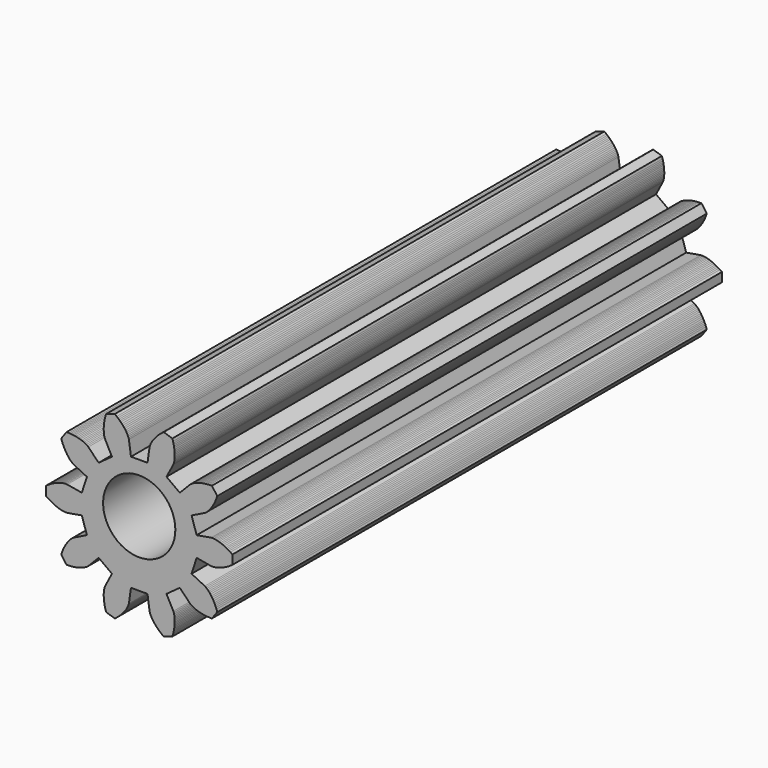
from build123d import *

# Parameters (mm, degrees)
F4_R     = 2.9504762809
F5_DEPTH = 250


# Not quite as in the source:
# - ends of sketch curves that miss each other by under 0.0002 mm in the source are joined


with BuildPart() as f3:
    # F0 (on Front) → F3 section 0
    with BuildSketch(Plane.XZ):
        with BuildLine():
            ThreePointArc((4.2753417889, -0.9237346066), (4.4837280553, -0.2822940953), (4.6921702972, 0.3591282284))
            Line((4.6921702972, 0.3591282284), (5.878934, 0.152889))
            Line((5.878934, 0.152889), (5.978914, 0.147897))
            Line((5.978914, 0.147897), (6.083031, 0.153397))
            Line((6.083031, 0.153397), (6.188792, 0.166293))
            Line((6.188792, 0.166293), (6.296123, 0.185564))
            Line((6.296123, 0.185564), (6.39688, 0.208667))
            Line((6.39688, 0.208667), (6.507485, 0.239158))
            Line((6.507485, 0.239158), (6.627466, 0.277934))
            Line((6.627466, 0.277934), (6.729844, 0.315505))
            Line((6.729844, 0.315505), (6.837582, 0.359366))
            Line((6.837582, 0.359366), (6.95036, 0.409935))
            Line((6.95036, 0.409935), (7.067828, 0.467611))
            Line((7.067828, 0.467611), (7.158791, 0.515766))
            Line((7.158791, 0.515766), (7.252025, 0.568292))
            Line((7.252025, 0.568292), (7.347362, 0.62534))
            Line((7.347362, 0.62534), (7.444626, 0.687056))
            Line((7.444626, 0.687056), (7.610854, 0.801339))
            Line((7.610854, 0.801339), (7.610854, 1.547781))
            Line((7.610854, 1.547781), (7.444624, 1.662064))
            Line((7.444624, 1.662064), (7.347361, 1.723779))
            Line((7.347361, 1.723779), (7.252025, 1.780827))
            Line((7.252025, 1.780827), (7.15879, 1.833354))
            Line((7.15879, 1.833354), (7.067828, 1.881508))
            Line((7.067828, 1.881508), (6.950358, 1.939185))
            Line((6.950358, 1.939185), (6.837582, 1.989753))
            Line((6.837582, 1.989753), (6.729843, 2.033614))
            Line((6.729843, 2.033614), (6.627464, 2.071186))
            Line((6.627464, 2.071186), (6.507485, 2.109962))
            Line((6.507485, 2.109962), (6.39688, 2.140452))
            Line((6.39688, 2.140452), (6.296123, 2.163555))
            Line((6.296123, 2.163555), (6.188792, 2.182826))
            Line((6.188792, 2.182826), (6.08303, 2.195722))
            Line((6.08303, 2.195722), (5.978914, 2.201222))
            Line((5.978914, 2.201222), (5.878933, 2.19623))
            Line((5.878933, 2.19623), (4.692172, 1.989989))
            ThreePointArc((4.692172, 1.989989), (4.4837309325, 2.6314120428), (4.2753451638, 3.2728530532))
            Line((4.2753451638, 3.2728530532), (5.35668, 3.80356))
            Line((5.35668, 3.80356), (5.4405, 3.858289))
            Line((5.4405, 3.858289), (5.5215, 3.923937))
            Line((5.5215, 3.923937), (5.599482, 3.996535))
            Line((5.599482, 3.996535), (5.674988, 4.075213))
            Line((5.674988, 4.075213), (5.742922, 4.153126))
            Line((5.742922, 4.153126), (5.814482, 4.242806))
            Line((5.814482, 4.242806), (5.888756, 4.344699))
            Line((5.888756, 4.344699), (5.949498, 4.435272))
            Line((5.949498, 4.435272), (6.010879, 4.534083))
            Line((6.010879, 4.534083), (6.072394, 4.641282))
            Line((6.072394, 4.641282), (6.133527, 4.75699))
            Line((6.133527, 4.75699), (6.178813, 4.849415))
            Line((6.178813, 4.849415), (6.223367, 4.946711))
            Line((6.223367, 4.946711), (6.266963, 5.048901))
            Line((6.266963, 5.048901), (6.309377, 5.156001))
            Line((6.309377, 5.156001), (6.376684, 5.346164))
            Line((6.376684, 5.346164), (5.937936, 5.950048))
            Line((5.937936, 5.950048), (5.73628, 5.944798))
            Line((5.73628, 5.944798), (5.621317, 5.937556))
            Line((5.621317, 5.937556), (5.510656, 5.927672))
            Line((5.510656, 5.927672), (5.404354, 5.915365))
            Line((5.404354, 5.915365), (5.302459, 5.900857))
            Line((5.302459, 5.900857), (5.173523, 5.878471))
            Line((5.173523, 5.878471), (5.052562, 5.853093))
            Line((5.052562, 5.853093), (4.939618, 5.825251))
            Line((4.939618, 5.825251), (4.834708, 5.79547))
            Line((4.834708, 5.79547), (4.714851, 5.756318))
            Line((4.714851, 5.756318), (4.607447, 5.715973))
            Line((4.607447, 5.715973), (4.512354, 5.67544))
            Line((4.512354, 5.67544), (4.414194, 5.627943))
            Line((4.414194, 5.627943), (4.321051, 5.576212))
            Line((4.321051, 5.576212), (4.233586, 5.519463))
            Line((4.233586, 5.519463), (4.155634, 5.456658))
            Line((4.155634, 5.456658), (3.31675, 4.592245))
            ThreePointArc((3.31675, 4.592245), (2.7710979645, 4.9886473644), (2.2254808469, 5.3850977893))
            Line((2.2254808469, 5.3850977893), (2.788358, 6.450042))
            Line((2.788358, 6.450042), (2.824001, 6.543587))
            Line((2.824001, 6.543587), (2.850944, 6.644307))
            Line((2.850944, 6.644307), (2.871361, 6.748877))
            Line((2.871361, 6.748877), (2.886201, 6.856911))
            Line((2.886201, 6.856911), (2.895364, 6.959874))
            Line((2.895364, 6.959874), (2.900545, 7.074489))
            Line((2.900545, 7.074489), (2.900742, 7.200579))
            Line((2.900742, 7.200579), (2.896647, 7.309556))
            Line((2.896647, 7.309556), (2.888225, 7.425575))
            Line((2.888225, 7.425575), (2.874982, 7.548459))
            Line((2.874982, 7.548459), (2.856428, 7.678002))
            Line((2.856428, 7.678002), (2.83874, 7.779394))
            Line((2.83874, 7.779394), (2.817595, 7.884296))
            Line((2.817595, 7.884296), (2.792799, 7.992596))
            Line((2.792799, 7.992596), (2.76416, 8.10417))
            Line((2.76416, 8.10417), (2.706839, 8.297578))
            Line((2.706839, 8.297578), (1.99693, 8.528241))
            Line((1.99693, 8.528241), (1.836873, 8.405463))
            Line((1.836873, 8.405463), (1.748122, 8.332031))
            Line((1.748122, 8.332031), (1.664405, 8.258989))
            Line((1.664405, 8.258989), (1.585639, 8.186549))
            Line((1.585639, 8.186549), (1.511732, 8.11492))
            Line((1.511732, 8.11492), (1.420578, 8.021022))
            Line((1.420578, 8.021022), (1.337635, 7.929392))
            Line((1.337635, 7.929392), (1.262627, 7.840481))
            Line((1.262627, 7.840481), (1.195258, 7.754723))
            Line((1.195258, 7.754723), (1.121305, 7.652599))
            Line((1.121305, 7.652599), (1.058128, 7.556829))
            Line((1.058128, 7.556829), (1.00502, 7.468143))
            Line((1.00502, 7.468143), (0.953525, 7.37202))
            Line((0.953525, 7.37202), (0.908577, 7.27542))
            Line((0.908577, 7.27542), (0.871173, 7.178099))
            Line((0.871173, 7.178099), (0.845025, 7.081469))
            Line((0.845025, 7.081469), (0.674443, 5.88906))
            ThreePointArc((0.674443, 5.88906), (1.5e-06, 5.8890320012), (-0.67444, 5.8890618078))
            Line((-0.67444, 5.8890618078), (-0.845022, 7.08147))
            Line((-0.845022, 7.08147), (-0.87117, 7.178099))
            Line((-0.87117, 7.178099), (-0.908574, 7.27542))
            Line((-0.908574, 7.27542), (-0.953521, 7.37202))
            Line((-0.953521, 7.37202), (-1.005016, 7.468143))
            Line((-1.005016, 7.468143), (-1.058124, 7.556829))
            Line((-1.058124, 7.556829), (-1.121301, 7.652598))
            Line((-1.121301, 7.652598), (-1.195255, 7.754725))
            Line((-1.195255, 7.754725), (-1.262624, 7.840481))
            Line((-1.262624, 7.840481), (-1.337632, 7.929392))
            Line((-1.337632, 7.929392), (-1.420575, 8.021024))
            Line((-1.420575, 8.021024), (-1.511728, 8.11492))
            Line((-1.511728, 8.11492), (-1.585636, 8.186551))
            Line((-1.585636, 8.186551), (-1.664402, 8.25899))
            Line((-1.664402, 8.25899), (-1.748119, 8.332032))
            Line((-1.748119, 8.332032), (-1.83687, 8.405464))
            Line((-1.83687, 8.405464), (-1.996926, 8.528241))
            Line((-1.996926, 8.528241), (-2.706835, 8.297578))
            Line((-2.706835, 8.297578), (-2.764157, 8.104169))
            Line((-2.764157, 8.104169), (-2.792795, 7.992595))
            Line((-2.792795, 7.992595), (-2.817591, 7.884296))
            Line((-2.817591, 7.884296), (-2.838736, 7.779392))
            Line((-2.838736, 7.779392), (-2.856425, 7.678002))
            Line((-2.856425, 7.678002), (-2.874978, 7.548459))
            Line((-2.874978, 7.548459), (-2.888221, 7.425576))
            Line((-2.888221, 7.425576), (-2.896643, 7.309556))
            Line((-2.896643, 7.309556), (-2.900739, 7.200578))
            Line((-2.900739, 7.200578), (-2.900542, 7.074489))
            Line((-2.900542, 7.074489), (-2.895361, 6.959875))
            Line((-2.895361, 6.959875), (-2.886197, 6.856911))
            Line((-2.886197, 6.856911), (-2.871358, 6.748877))
            Line((-2.871358, 6.748877), (-2.850941, 6.644307))
            Line((-2.850941, 6.644307), (-2.823998, 6.543587))
            Line((-2.823998, 6.543587), (-2.788355, 6.450042))
            Line((-2.788355, 6.450042), (-2.225478, 5.385097))
            ThreePointArc((-2.225478, 5.385097), (-2.771095971, 4.9886482498), (-3.3167477562, 4.592246041))
            Line((-3.3167477562, 4.592246041), (-4.155632, 5.456658))
            Line((-4.155632, 5.456658), (-4.233584, 5.519464))
            Line((-4.233584, 5.519464), (-4.321049, 5.576213))
            Line((-4.321049, 5.576213), (-4.414192, 5.627944))
            Line((-4.414192, 5.627944), (-4.512352, 5.675442))
            Line((-4.512352, 5.675442), (-4.607445, 5.715974))
            Line((-4.607445, 5.715974), (-4.714848, 5.756319))
            Line((-4.714848, 5.756319), (-4.834706, 5.795471))
            Line((-4.834706, 5.795471), (-4.939616, 5.825252))
            Line((-4.939616, 5.825252), (-5.052559, 5.853094))
            Line((-5.052559, 5.853094), (-5.173522, 5.878472))
            Line((-5.173522, 5.878472), (-5.302457, 5.900857))
            Line((-5.302457, 5.900857), (-5.404352, 5.915366))
            Line((-5.404352, 5.915366), (-5.510654, 5.927673))
            Line((-5.510654, 5.927673), (-5.621316, 5.937558))
            Line((-5.621316, 5.937558), (-5.736279, 5.944799))
            Line((-5.736279, 5.944799), (-5.937934, 5.950049))
            Line((-5.937934, 5.950049), (-6.376683, 5.346165))
            Line((-6.376683, 5.346165), (-6.309373, 5.156001))
            Line((-6.309373, 5.156001), (-6.266961, 5.048902))
            Line((-6.266961, 5.048902), (-6.223364, 4.946712))
            Line((-6.223364, 4.946712), (-6.17881, 4.849415))
            Line((-6.17881, 4.849415), (-6.133525, 4.756991))
            Line((-6.133525, 4.756991), (-6.072391, 4.641283))
            Line((-6.072391, 4.641283), (-6.010877, 4.534084))
            Line((-6.010877, 4.534084), (-5.949495, 4.435272))
            Line((-5.949495, 4.435272), (-5.888753, 4.344699))
            Line((-5.888753, 4.344699), (-5.81448, 4.242807))
            Line((-5.81448, 4.242807), (-5.74292, 4.153128))
            Line((-5.74292, 4.153128), (-5.674986, 4.075214))
            Line((-5.674986, 4.075214), (-5.59948, 3.996536))
            Line((-5.59948, 3.996536), (-5.521498, 3.923937))
            Line((-5.521498, 3.923937), (-5.440498, 3.85829))
            Line((-5.440498, 3.85829), (-5.356678, 3.803561))
            Line((-5.356678, 3.803561), (-4.275343, 3.272853))
            ThreePointArc((-4.275343, 3.272853), (-4.4837282639, 2.6314121631), (-4.6921703347, 1.9899897838))
            Line((-4.6921703347, 1.9899897838), (-5.878932, 2.196231))
            Line((-5.878932, 2.196231), (-5.978913, 2.201222))
            Line((-5.978913, 2.201222), (-6.08303, 2.195723))
            Line((-6.08303, 2.195723), (-6.188791, 2.182826))
            Line((-6.188791, 2.182826), (-6.296122, 2.163555))
            Line((-6.296122, 2.163555), (-6.396879, 2.140453))
            Line((-6.396879, 2.140453), (-6.507485, 2.109962))
            Line((-6.507485, 2.109962), (-6.627465, 2.071186))
            Line((-6.627465, 2.071186), (-6.729843, 2.033615))
            Line((-6.729843, 2.033615), (-6.837581, 1.989753))
            Line((-6.837581, 1.989753), (-6.950359, 1.939185))
            Line((-6.950359, 1.939185), (-7.067828, 1.881509))
            Line((-7.067828, 1.881509), (-7.158791, 1.833354))
            Line((-7.158791, 1.833354), (-7.252025, 1.780828))
            Line((-7.252025, 1.780828), (-7.347361, 1.723779))
            Line((-7.347361, 1.723779), (-7.444625, 1.662064))
            Line((-7.444625, 1.662064), (-7.610853, 1.547781))
            Line((-7.610853, 1.547781), (-7.610853, 0.801339))
            Line((-7.610853, 0.801339), (-7.444624, 0.687056))
            Line((-7.444624, 0.687056), (-7.34736, 0.625341))
            Line((-7.34736, 0.625341), (-7.252024, 0.568293))
            Line((-7.252024, 0.568293), (-7.158789, 0.515766))
            Line((-7.158789, 0.515766), (-7.067828, 0.467612))
            Line((-7.067828, 0.467612), (-6.950358, 0.409935))
            Line((-6.950358, 0.409935), (-6.837581, 0.359367))
            Line((-6.837581, 0.359367), (-6.729843, 0.315506))
            Line((-6.729843, 0.315506), (-6.627464, 0.277934))
            Line((-6.627464, 0.277934), (-6.507485, 0.239159))
            Line((-6.507485, 0.239159), (-6.396879, 0.208668))
            Line((-6.396879, 0.208668), (-6.296122, 0.185565))
            Line((-6.296122, 0.185565), (-6.18879, 0.166294))
            Line((-6.18879, 0.166294), (-6.083029, 0.153398))
            Line((-6.083029, 0.153398), (-5.978913, 0.147898))
            Line((-5.978913, 0.147898), (-5.878932, 0.15289))
            Line((-5.878932, 0.15289), (-4.692171, 0.359131))
            ThreePointArc((-4.692171, 0.359131), (-4.4837298858, -0.2822915276), (-4.2753442362, -0.9237320767))
            Line((-4.2753442362, -0.9237320767), (-5.356681, -1.45444))
            Line((-5.356681, -1.45444), (-5.440501, -1.509168))
            Line((-5.440501, -1.509168), (-5.5215, -1.574816))
            Line((-5.5215, -1.574816), (-5.599482, -1.647414))
            Line((-5.599482, -1.647414), (-5.674988, -1.726092))
            Line((-5.674988, -1.726092), (-5.742923, -1.804005))
            Line((-5.742923, -1.804005), (-5.814482, -1.893685))
            Line((-5.814482, -1.893685), (-5.888757, -1.995578))
            Line((-5.888757, -1.995578), (-5.949499, -2.08615))
            Line((-5.949499, -2.08615), (-6.010879, -2.184962))
            Line((-6.010879, -2.184962), (-6.072395, -2.292162))
            Line((-6.072395, -2.292162), (-6.133528, -2.407869))
            Line((-6.133528, -2.407869), (-6.178814, -2.500294))
            Line((-6.178814, -2.500294), (-6.223368, -2.59759))
            Line((-6.223368, -2.59759), (-6.266964, -2.69978))
            Line((-6.266964, -2.69978), (-6.309378, -2.80688))
            Line((-6.309378, -2.80688), (-6.376685, -2.997043))
            Line((-6.376685, -2.997043), (-5.937937, -3.600927))
            Line((-5.937937, -3.600927), (-5.736281, -3.595677))
            Line((-5.736281, -3.595677), (-5.621318, -3.588435))
            Line((-5.621318, -3.588435), (-5.510657, -3.578551))
            Line((-5.510657, -3.578551), (-5.404354, -3.566244))
            Line((-5.404354, -3.566244), (-5.30246, -3.551736))
            Line((-5.30246, -3.551736), (-5.173523, -3.52935))
            Line((-5.173523, -3.52935), (-5.052562, -3.503972))
            Line((-5.052562, -3.503972), (-4.939619, -3.47613))
            Line((-4.939619, -3.47613), (-4.834708, -3.446349))
            Line((-4.834708, -3.446349), (-4.714851, -3.407198))
            Line((-4.714851, -3.407198), (-4.607448, -3.366853))
            Line((-4.607448, -3.366853), (-4.512355, -3.32632))
            Line((-4.512355, -3.32632), (-4.414194, -3.278822))
            Line((-4.414194, -3.278822), (-4.321052, -3.227091))
            Line((-4.321052, -3.227091), (-4.233587, -3.170342))
            Line((-4.233587, -3.170342), (-4.155635, -3.107537))
            Line((-4.155635, -3.107537), (-3.31675, -2.243124))
            ThreePointArc((-3.31675, -2.243124), (-2.7710983472, -2.6395268912), (-2.2254812543, -3.0359773499))
            Line((-2.2254812543, -3.0359773499), (-2.788359, -4.100922))
            Line((-2.788359, -4.100922), (-2.824002, -4.194467))
            Line((-2.824002, -4.194467), (-2.850945, -4.295187))
            Line((-2.850945, -4.295187), (-2.871362, -4.399757))
            Line((-2.871362, -4.399757), (-2.886201, -4.50779))
            Line((-2.886201, -4.50779), (-2.895365, -4.610754))
            Line((-2.895365, -4.610754), (-2.900546, -4.725369))
            Line((-2.900546, -4.725369), (-2.900744, -4.851459))
            Line((-2.900744, -4.851459), (-2.896648, -4.960437))
            Line((-2.896648, -4.960437), (-2.888226, -5.076456))
            Line((-2.888226, -5.076456), (-2.874983, -5.19934))
            Line((-2.874983, -5.19934), (-2.856429, -5.328883))
            Line((-2.856429, -5.328883), (-2.838741, -5.430275))
            Line((-2.838741, -5.430275), (-2.817596, -5.535177))
            Line((-2.817596, -5.535177), (-2.7928, -5.643476))
            Line((-2.7928, -5.643476), (-2.764162, -5.75505))
            Line((-2.764162, -5.75505), (-2.70684, -5.948458))
            Line((-2.70684, -5.948458), (-1.996931, -6.179121))
            Line((-1.996931, -6.179121), (-1.836874, -6.056343))
            Line((-1.836874, -6.056343), (-1.748123, -5.982912))
            Line((-1.748123, -5.982912), (-1.664406, -5.90987))
            Line((-1.664406, -5.90987), (-1.585639, -5.83743))
            Line((-1.585639, -5.83743), (-1.511733, -5.765801))
            Line((-1.511733, -5.765801), (-1.420579, -5.671903))
            Line((-1.420579, -5.671903), (-1.337636, -5.580273))
            Line((-1.337636, -5.580273), (-1.262628, -5.491361))
            Line((-1.262628, -5.491361), (-1.195259, -5.405603))
            Line((-1.195259, -5.405603), (-1.121305, -5.303479))
            Line((-1.121305, -5.303479), (-1.058128, -5.207709))
            Line((-1.058128, -5.207709), (-1.00502, -5.119023))
            Line((-1.00502, -5.119023), (-0.953526, -5.0229))
            Line((-0.953526, -5.0229), (-0.908578, -4.9263))
            Line((-0.908578, -4.9263), (-0.871174, -4.828979))
            Line((-0.871174, -4.828979), (-0.845026, -4.73235))
            Line((-0.845026, -4.73235), (-0.674443, -3.539941))
            ThreePointArc((-0.674443, -3.539941), (-1.5e-06, -3.5399120003), (0.67444, -3.5399416176))
            Line((0.67444, -3.5399416176), (0.845021, -4.732351))
            Line((0.845021, -4.732351), (0.87117, -4.82898))
            Line((0.87117, -4.82898), (0.908574, -4.926302))
            Line((0.908574, -4.926302), (0.953521, -5.022901))
            Line((0.953521, -5.022901), (1.005016, -5.119024))
            Line((1.005016, -5.119024), (1.058123, -5.20771))
            Line((1.058123, -5.20771), (1.1213, -5.30348))
            Line((1.1213, -5.30348), (1.195254, -5.405606))
            Line((1.195254, -5.405606), (1.262623, -5.491364))
            Line((1.262623, -5.491364), (1.337631, -5.580275))
            Line((1.337631, -5.580275), (1.420574, -5.671906))
            Line((1.420574, -5.671906), (1.511728, -5.765803))
            Line((1.511728, -5.765803), (1.585635, -5.837433))
            Line((1.585635, -5.837433), (1.664401, -5.909872))
            Line((1.664401, -5.909872), (1.748118, -5.982913))
            Line((1.748118, -5.982913), (1.836869, -6.056346))
            Line((1.836869, -6.056346), (1.996925, -6.179123))
            Line((1.996925, -6.179123), (2.706834, -5.94846))
            Line((2.706834, -5.94846), (2.764156, -5.755051))
            Line((2.764156, -5.755051), (2.792795, -5.643476))
            Line((2.792795, -5.643476), (2.817591, -5.535178))
            Line((2.817591, -5.535178), (2.838735, -5.430275))
            Line((2.838735, -5.430275), (2.856424, -5.328885))
            Line((2.856424, -5.328885), (2.874977, -5.199341))
            Line((2.874977, -5.199341), (2.888221, -5.076458))
            Line((2.888221, -5.076458), (2.896643, -4.960438))
            Line((2.896643, -4.960438), (2.900738, -4.851459))
            Line((2.900738, -4.851459), (2.900541, -4.725371))
            Line((2.900541, -4.725371), (2.89536, -4.610756))
            Line((2.89536, -4.610756), (2.886197, -4.507792))
            Line((2.886197, -4.507792), (2.871357, -4.399759))
            Line((2.871357, -4.399759), (2.850941, -4.295188))
            Line((2.850941, -4.295188), (2.823998, -4.194468))
            Line((2.823998, -4.194468), (2.788354, -4.100924))
            Line((2.788354, -4.100924), (2.225479, -3.035979))
            ThreePointArc((2.225479, -3.035979), (2.7710963565, -2.6395289039), (3.3167481995, -2.2431262746))
            Line((3.3167481995, -2.2431262746), (4.155631, -3.10754))
            Line((4.155631, -3.10754), (4.233583, -3.170346))
            Line((4.233583, -3.170346), (4.321048, -3.227095))
            Line((4.321048, -3.227095), (4.41419, -3.278826))
            Line((4.41419, -3.278826), (4.51235, -3.326324))
            Line((4.51235, -3.326324), (4.607444, -3.366856))
            Line((4.607444, -3.366856), (4.714847, -3.407201))
            Line((4.714847, -3.407201), (4.834705, -3.446354))
            Line((4.834705, -3.446354), (4.939615, -3.476134))
            Line((4.939615, -3.476134), (5.052558, -3.503976))
            Line((5.052558, -3.503976), (5.17352, -3.529355))
            Line((5.17352, -3.529355), (5.302456, -3.55174))
            Line((5.302456, -3.55174), (5.404351, -3.566249))
            Line((5.404351, -3.566249), (5.510653, -3.578556))
            Line((5.510653, -3.578556), (5.621314, -3.58844))
            Line((5.621314, -3.58844), (5.736278, -3.595682))
            Line((5.736278, -3.595682), (5.937933, -3.600932))
            Line((5.937933, -3.600932), (6.376681, -2.997048))
            Line((6.376681, -2.997048), (6.309372, -2.806883))
            Line((6.309372, -2.806883), (6.26696, -2.699785))
            Line((6.26696, -2.699785), (6.223363, -2.597595))
            Line((6.223363, -2.597595), (6.178809, -2.500297))
            Line((6.178809, -2.500297), (6.133524, -2.407874))
            Line((6.133524, -2.407874), (6.07239, -2.292165))
            Line((6.07239, -2.292165), (6.010875, -2.184966))
            Line((6.010875, -2.184966), (5.949495, -2.086155))
            Line((5.949495, -2.086155), (5.888752, -1.995582))
            Line((5.888752, -1.995582), (5.814479, -1.89369))
            Line((5.814479, -1.89369), (5.742919, -1.80401))
            Line((5.742919, -1.80401), (5.674985, -1.726096))
            Line((5.674985, -1.726096), (5.599479, -1.647418))
            Line((5.599479, -1.647418), (5.521497, -1.574819))
            Line((5.521497, -1.574819), (5.440498, -1.509172))
            Line((5.440498, -1.509172), (5.356677, -1.454443))
            Line((5.356677, -1.454443), (4.2753417889, -0.9237346066))
        make_face()
    # F2 (on offset) → F3 section 1
    with BuildSketch(Plane.XZ.offset(50)):
        with BuildLine():
            ThreePointArc((4.2753417889, -0.9237346066), (4.4837280553, -0.2822940953), (4.6921702972, 0.3591282284))
            Line((4.6921702972, 0.3591282284), (5.878934, 0.152889))
            Line((5.878934, 0.152889), (5.978914, 0.147897))
            Line((5.978914, 0.147897), (6.083031, 0.153397))
            Line((6.083031, 0.153397), (6.188792, 0.166293))
            Line((6.188792, 0.166293), (6.296123, 0.185564))
            Line((6.296123, 0.185564), (6.39688, 0.208667))
            Line((6.39688, 0.208667), (6.507485, 0.239158))
            Line((6.507485, 0.239158), (6.627466, 0.277934))
            Line((6.627466, 0.277934), (6.729844, 0.315505))
            Line((6.729844, 0.315505), (6.837582, 0.359366))
            Line((6.837582, 0.359366), (6.95036, 0.409935))
            Line((6.95036, 0.409935), (7.067828, 0.467611))
            Line((7.067828, 0.467611), (7.158791, 0.515766))
            Line((7.158791, 0.515766), (7.252025, 0.568292))
            Line((7.252025, 0.568292), (7.347362, 0.62534))
            Line((7.347362, 0.62534), (7.444626, 0.687056))
            Line((7.444626, 0.687056), (7.610854, 0.801339))
            Line((7.610854, 0.801339), (7.610854, 1.547781))
            Line((7.610854, 1.547781), (7.444624, 1.662064))
            Line((7.444624, 1.662064), (7.347361, 1.723779))
            Line((7.347361, 1.723779), (7.252025, 1.780827))
            Line((7.252025, 1.780827), (7.15879, 1.833354))
            Line((7.15879, 1.833354), (7.067828, 1.881508))
            Line((7.067828, 1.881508), (6.950358, 1.939185))
            Line((6.950358, 1.939185), (6.837582, 1.989753))
            Line((6.837582, 1.989753), (6.729843, 2.033614))
            Line((6.729843, 2.033614), (6.627464, 2.071186))
            Line((6.627464, 2.071186), (6.507485, 2.109962))
            Line((6.507485, 2.109962), (6.39688, 2.140452))
            Line((6.39688, 2.140452), (6.296123, 2.163555))
            Line((6.296123, 2.163555), (6.188792, 2.182826))
            Line((6.188792, 2.182826), (6.08303, 2.195722))
            Line((6.08303, 2.195722), (5.978914, 2.201222))
            Line((5.978914, 2.201222), (5.878933, 2.19623))
            Line((5.878933, 2.19623), (4.692172, 1.989989))
            ThreePointArc((4.692172, 1.989989), (4.4837309325, 2.6314120428), (4.2753451638, 3.2728530532))
            Line((4.2753451638, 3.2728530532), (5.35668, 3.80356))
            Line((5.35668, 3.80356), (5.4405, 3.858289))
            Line((5.4405, 3.858289), (5.5215, 3.923937))
            Line((5.5215, 3.923937), (5.599482, 3.996535))
            Line((5.599482, 3.996535), (5.674988, 4.075213))
            Line((5.674988, 4.075213), (5.742922, 4.153126))
            Line((5.742922, 4.153126), (5.814482, 4.242806))
            Line((5.814482, 4.242806), (5.888756, 4.344699))
            Line((5.888756, 4.344699), (5.949498, 4.435272))
            Line((5.949498, 4.435272), (6.010879, 4.534083))
            Line((6.010879, 4.534083), (6.072394, 4.641282))
            Line((6.072394, 4.641282), (6.133527, 4.75699))
            Line((6.133527, 4.75699), (6.178813, 4.849415))
            Line((6.178813, 4.849415), (6.223367, 4.946711))
            Line((6.223367, 4.946711), (6.266963, 5.048901))
            Line((6.266963, 5.048901), (6.309377, 5.156001))
            Line((6.309377, 5.156001), (6.376684, 5.346164))
            Line((6.376684, 5.346164), (5.937936, 5.950048))
            Line((5.937936, 5.950048), (5.73628, 5.944798))
            Line((5.73628, 5.944798), (5.621317, 5.937556))
            Line((5.621317, 5.937556), (5.510656, 5.927672))
            Line((5.510656, 5.927672), (5.404354, 5.915365))
            Line((5.404354, 5.915365), (5.302459, 5.900857))
            Line((5.302459, 5.900857), (5.173523, 5.878471))
            Line((5.173523, 5.878471), (5.052562, 5.853093))
            Line((5.052562, 5.853093), (4.939618, 5.825251))
            Line((4.939618, 5.825251), (4.834708, 5.79547))
            Line((4.834708, 5.79547), (4.714851, 5.756318))
            Line((4.714851, 5.756318), (4.607447, 5.715973))
            Line((4.607447, 5.715973), (4.512354, 5.67544))
            Line((4.512354, 5.67544), (4.414194, 5.627943))
            Line((4.414194, 5.627943), (4.321051, 5.576212))
            Line((4.321051, 5.576212), (4.233586, 5.519463))
            Line((4.233586, 5.519463), (4.155634, 5.456658))
            Line((4.155634, 5.456658), (3.31675, 4.592245))
            ThreePointArc((3.31675, 4.592245), (2.7710979645, 4.9886473644), (2.2254808469, 5.3850977893))
            Line((2.2254808469, 5.3850977893), (2.788358, 6.450042))
            Line((2.788358, 6.450042), (2.824001, 6.543587))
            Line((2.824001, 6.543587), (2.850944, 6.644307))
            Line((2.850944, 6.644307), (2.871361, 6.748877))
            Line((2.871361, 6.748877), (2.886201, 6.856911))
            Line((2.886201, 6.856911), (2.895364, 6.959874))
            Line((2.895364, 6.959874), (2.900545, 7.074489))
            Line((2.900545, 7.074489), (2.900742, 7.200579))
            Line((2.900742, 7.200579), (2.896647, 7.309556))
            Line((2.896647, 7.309556), (2.888225, 7.425575))
            Line((2.888225, 7.425575), (2.874982, 7.548459))
            Line((2.874982, 7.548459), (2.856428, 7.678002))
            Line((2.856428, 7.678002), (2.83874, 7.779394))
            Line((2.83874, 7.779394), (2.817595, 7.884296))
            Line((2.817595, 7.884296), (2.792799, 7.992596))
            Line((2.792799, 7.992596), (2.76416, 8.10417))
            Line((2.76416, 8.10417), (2.706839, 8.297578))
            Line((2.706839, 8.297578), (1.99693, 8.528241))
            Line((1.99693, 8.528241), (1.836873, 8.405463))
            Line((1.836873, 8.405463), (1.748122, 8.332031))
            Line((1.748122, 8.332031), (1.664405, 8.258989))
            Line((1.664405, 8.258989), (1.585639, 8.186549))
            Line((1.585639, 8.186549), (1.511732, 8.11492))
            Line((1.511732, 8.11492), (1.420578, 8.021022))
            Line((1.420578, 8.021022), (1.337635, 7.929392))
            Line((1.337635, 7.929392), (1.262627, 7.840481))
            Line((1.262627, 7.840481), (1.195258, 7.754723))
            Line((1.195258, 7.754723), (1.121305, 7.652599))
            Line((1.121305, 7.652599), (1.058128, 7.556829))
            Line((1.058128, 7.556829), (1.00502, 7.468143))
            Line((1.00502, 7.468143), (0.953525, 7.37202))
            Line((0.953525, 7.37202), (0.908577, 7.27542))
            Line((0.908577, 7.27542), (0.871173, 7.178099))
            Line((0.871173, 7.178099), (0.845025, 7.081469))
            Line((0.845025, 7.081469), (0.674443, 5.88906))
            ThreePointArc((0.674443, 5.88906), (1.5e-06, 5.8890320012), (-0.67444, 5.8890618078))
            Line((-0.67444, 5.8890618078), (-0.845022, 7.08147))
            Line((-0.845022, 7.08147), (-0.87117, 7.178099))
            Line((-0.87117, 7.178099), (-0.908574, 7.27542))
            Line((-0.908574, 7.27542), (-0.953521, 7.37202))
            Line((-0.953521, 7.37202), (-1.005016, 7.468143))
            Line((-1.005016, 7.468143), (-1.058124, 7.556829))
            Line((-1.058124, 7.556829), (-1.121301, 7.652598))
            Line((-1.121301, 7.652598), (-1.195255, 7.754725))
            Line((-1.195255, 7.754725), (-1.262624, 7.840481))
            Line((-1.262624, 7.840481), (-1.337632, 7.929392))
            Line((-1.337632, 7.929392), (-1.420575, 8.021024))
            Line((-1.420575, 8.021024), (-1.511728, 8.11492))
            Line((-1.511728, 8.11492), (-1.585636, 8.186551))
            Line((-1.585636, 8.186551), (-1.664402, 8.25899))
            Line((-1.664402, 8.25899), (-1.748119, 8.332032))
            Line((-1.748119, 8.332032), (-1.83687, 8.405464))
            Line((-1.83687, 8.405464), (-1.996926, 8.528241))
            Line((-1.996926, 8.528241), (-2.706835, 8.297578))
            Line((-2.706835, 8.297578), (-2.764157, 8.104169))
            Line((-2.764157, 8.104169), (-2.792795, 7.992595))
            Line((-2.792795, 7.992595), (-2.817591, 7.884296))
            Line((-2.817591, 7.884296), (-2.838736, 7.779392))
            Line((-2.838736, 7.779392), (-2.856425, 7.678002))
            Line((-2.856425, 7.678002), (-2.874978, 7.548459))
            Line((-2.874978, 7.548459), (-2.888221, 7.425576))
            Line((-2.888221, 7.425576), (-2.896643, 7.309556))
            Line((-2.896643, 7.309556), (-2.900739, 7.200578))
            Line((-2.900739, 7.200578), (-2.900542, 7.074489))
            Line((-2.900542, 7.074489), (-2.895361, 6.959875))
            Line((-2.895361, 6.959875), (-2.886197, 6.856911))
            Line((-2.886197, 6.856911), (-2.871358, 6.748877))
            Line((-2.871358, 6.748877), (-2.850941, 6.644307))
            Line((-2.850941, 6.644307), (-2.823998, 6.543587))
            Line((-2.823998, 6.543587), (-2.788355, 6.450042))
            Line((-2.788355, 6.450042), (-2.225478, 5.385097))
            ThreePointArc((-2.225478, 5.385097), (-2.771095971, 4.9886482498), (-3.3167477562, 4.592246041))
            Line((-3.3167477562, 4.592246041), (-4.155632, 5.456658))
            Line((-4.155632, 5.456658), (-4.233584, 5.519464))
            Line((-4.233584, 5.519464), (-4.321049, 5.576213))
            Line((-4.321049, 5.576213), (-4.414192, 5.627944))
            Line((-4.414192, 5.627944), (-4.512352, 5.675442))
            Line((-4.512352, 5.675442), (-4.607445, 5.715974))
            Line((-4.607445, 5.715974), (-4.714848, 5.756319))
            Line((-4.714848, 5.756319), (-4.834706, 5.795471))
            Line((-4.834706, 5.795471), (-4.939616, 5.825252))
            Line((-4.939616, 5.825252), (-5.052559, 5.853094))
            Line((-5.052559, 5.853094), (-5.173522, 5.878472))
            Line((-5.173522, 5.878472), (-5.302457, 5.900857))
            Line((-5.302457, 5.900857), (-5.404352, 5.915366))
            Line((-5.404352, 5.915366), (-5.510654, 5.927673))
            Line((-5.510654, 5.927673), (-5.621316, 5.937558))
            Line((-5.621316, 5.937558), (-5.736279, 5.944799))
            Line((-5.736279, 5.944799), (-5.937934, 5.950049))
            Line((-5.937934, 5.950049), (-6.376683, 5.346165))
            Line((-6.376683, 5.346165), (-6.309373, 5.156001))
            Line((-6.309373, 5.156001), (-6.266961, 5.048902))
            Line((-6.266961, 5.048902), (-6.223364, 4.946712))
            Line((-6.223364, 4.946712), (-6.17881, 4.849415))
            Line((-6.17881, 4.849415), (-6.133525, 4.756991))
            Line((-6.133525, 4.756991), (-6.072391, 4.641283))
            Line((-6.072391, 4.641283), (-6.010877, 4.534084))
            Line((-6.010877, 4.534084), (-5.949495, 4.435272))
            Line((-5.949495, 4.435272), (-5.888753, 4.344699))
            Line((-5.888753, 4.344699), (-5.81448, 4.242807))
            Line((-5.81448, 4.242807), (-5.74292, 4.153128))
            Line((-5.74292, 4.153128), (-5.674986, 4.075214))
            Line((-5.674986, 4.075214), (-5.59948, 3.996536))
            Line((-5.59948, 3.996536), (-5.521498, 3.923937))
            Line((-5.521498, 3.923937), (-5.440498, 3.85829))
            Line((-5.440498, 3.85829), (-5.356678, 3.803561))
            Line((-5.356678, 3.803561), (-4.275343, 3.272853))
            ThreePointArc((-4.275343, 3.272853), (-4.4837282639, 2.6314121631), (-4.6921703347, 1.9899897838))
            Line((-4.6921703347, 1.9899897838), (-5.878932, 2.196231))
            Line((-5.878932, 2.196231), (-5.978913, 2.201222))
            Line((-5.978913, 2.201222), (-6.08303, 2.195723))
            Line((-6.08303, 2.195723), (-6.188791, 2.182826))
            Line((-6.188791, 2.182826), (-6.296122, 2.163555))
            Line((-6.296122, 2.163555), (-6.396879, 2.140453))
            Line((-6.396879, 2.140453), (-6.507485, 2.109962))
            Line((-6.507485, 2.109962), (-6.627465, 2.071186))
            Line((-6.627465, 2.071186), (-6.729843, 2.033615))
            Line((-6.729843, 2.033615), (-6.837581, 1.989753))
            Line((-6.837581, 1.989753), (-6.950359, 1.939185))
            Line((-6.950359, 1.939185), (-7.067828, 1.881509))
            Line((-7.067828, 1.881509), (-7.158791, 1.833354))
            Line((-7.158791, 1.833354), (-7.252025, 1.780828))
            Line((-7.252025, 1.780828), (-7.347361, 1.723779))
            Line((-7.347361, 1.723779), (-7.444625, 1.662064))
            Line((-7.444625, 1.662064), (-7.610853, 1.547781))
            Line((-7.610853, 1.547781), (-7.610853, 0.801339))
            Line((-7.610853, 0.801339), (-7.444624, 0.687056))
            Line((-7.444624, 0.687056), (-7.34736, 0.625341))
            Line((-7.34736, 0.625341), (-7.252024, 0.568293))
            Line((-7.252024, 0.568293), (-7.158789, 0.515766))
            Line((-7.158789, 0.515766), (-7.067828, 0.467612))
            Line((-7.067828, 0.467612), (-6.950358, 0.409935))
            Line((-6.950358, 0.409935), (-6.837581, 0.359367))
            Line((-6.837581, 0.359367), (-6.729843, 0.315506))
            Line((-6.729843, 0.315506), (-6.627464, 0.277934))
            Line((-6.627464, 0.277934), (-6.507485, 0.239159))
            Line((-6.507485, 0.239159), (-6.396879, 0.208668))
            Line((-6.396879, 0.208668), (-6.296122, 0.185565))
            Line((-6.296122, 0.185565), (-6.18879, 0.166294))
            Line((-6.18879, 0.166294), (-6.083029, 0.153398))
            Line((-6.083029, 0.153398), (-5.978913, 0.147898))
            Line((-5.978913, 0.147898), (-5.878932, 0.15289))
            Line((-5.878932, 0.15289), (-4.692171, 0.359131))
            ThreePointArc((-4.692171, 0.359131), (-4.4837298858, -0.2822915276), (-4.2753442362, -0.9237320767))
            Line((-4.2753442362, -0.9237320767), (-5.356681, -1.45444))
            Line((-5.356681, -1.45444), (-5.440501, -1.509168))
            Line((-5.440501, -1.509168), (-5.5215, -1.574816))
            Line((-5.5215, -1.574816), (-5.599482, -1.647414))
            Line((-5.599482, -1.647414), (-5.674988, -1.726092))
            Line((-5.674988, -1.726092), (-5.742923, -1.804005))
            Line((-5.742923, -1.804005), (-5.814482, -1.893685))
            Line((-5.814482, -1.893685), (-5.888757, -1.995578))
            Line((-5.888757, -1.995578), (-5.949499, -2.08615))
            Line((-5.949499, -2.08615), (-6.010879, -2.184962))
            Line((-6.010879, -2.184962), (-6.072395, -2.292162))
            Line((-6.072395, -2.292162), (-6.133528, -2.407869))
            Line((-6.133528, -2.407869), (-6.178814, -2.500294))
            Line((-6.178814, -2.500294), (-6.223368, -2.59759))
            Line((-6.223368, -2.59759), (-6.266964, -2.69978))
            Line((-6.266964, -2.69978), (-6.309378, -2.80688))
            Line((-6.309378, -2.80688), (-6.376685, -2.997043))
            Line((-6.376685, -2.997043), (-5.937937, -3.600927))
            Line((-5.937937, -3.600927), (-5.736281, -3.595677))
            Line((-5.736281, -3.595677), (-5.621318, -3.588435))
            Line((-5.621318, -3.588435), (-5.510657, -3.578551))
            Line((-5.510657, -3.578551), (-5.404354, -3.566244))
            Line((-5.404354, -3.566244), (-5.30246, -3.551736))
            Line((-5.30246, -3.551736), (-5.173523, -3.52935))
            Line((-5.173523, -3.52935), (-5.052562, -3.503972))
            Line((-5.052562, -3.503972), (-4.939619, -3.47613))
            Line((-4.939619, -3.47613), (-4.834708, -3.446349))
            Line((-4.834708, -3.446349), (-4.714851, -3.407198))
            Line((-4.714851, -3.407198), (-4.607448, -3.366853))
            Line((-4.607448, -3.366853), (-4.512355, -3.32632))
            Line((-4.512355, -3.32632), (-4.414194, -3.278822))
            Line((-4.414194, -3.278822), (-4.321052, -3.227091))
            Line((-4.321052, -3.227091), (-4.233587, -3.170342))
            Line((-4.233587, -3.170342), (-4.155635, -3.107537))
            Line((-4.155635, -3.107537), (-3.31675, -2.243124))
            ThreePointArc((-3.31675, -2.243124), (-2.7710983472, -2.6395268912), (-2.2254812543, -3.0359773499))
            Line((-2.2254812543, -3.0359773499), (-2.788359, -4.100922))
            Line((-2.788359, -4.100922), (-2.824002, -4.194467))
            Line((-2.824002, -4.194467), (-2.850945, -4.295187))
            Line((-2.850945, -4.295187), (-2.871362, -4.399757))
            Line((-2.871362, -4.399757), (-2.886201, -4.50779))
            Line((-2.886201, -4.50779), (-2.895365, -4.610754))
            Line((-2.895365, -4.610754), (-2.900546, -4.725369))
            Line((-2.900546, -4.725369), (-2.900744, -4.851459))
            Line((-2.900744, -4.851459), (-2.896648, -4.960437))
            Line((-2.896648, -4.960437), (-2.888226, -5.076456))
            Line((-2.888226, -5.076456), (-2.874983, -5.19934))
            Line((-2.874983, -5.19934), (-2.856429, -5.328883))
            Line((-2.856429, -5.328883), (-2.838741, -5.430275))
            Line((-2.838741, -5.430275), (-2.817596, -5.535177))
            Line((-2.817596, -5.535177), (-2.7928, -5.643476))
            Line((-2.7928, -5.643476), (-2.764162, -5.75505))
            Line((-2.764162, -5.75505), (-2.70684, -5.948458))
            Line((-2.70684, -5.948458), (-1.996931, -6.179121))
            Line((-1.996931, -6.179121), (-1.836874, -6.056343))
            Line((-1.836874, -6.056343), (-1.748123, -5.982912))
            Line((-1.748123, -5.982912), (-1.664406, -5.90987))
            Line((-1.664406, -5.90987), (-1.585639, -5.83743))
            Line((-1.585639, -5.83743), (-1.511733, -5.765801))
            Line((-1.511733, -5.765801), (-1.420579, -5.671903))
            Line((-1.420579, -5.671903), (-1.337636, -5.580273))
            Line((-1.337636, -5.580273), (-1.262628, -5.491361))
            Line((-1.262628, -5.491361), (-1.195259, -5.405603))
            Line((-1.195259, -5.405603), (-1.121305, -5.303479))
            Line((-1.121305, -5.303479), (-1.058128, -5.207709))
            Line((-1.058128, -5.207709), (-1.00502, -5.119023))
            Line((-1.00502, -5.119023), (-0.953526, -5.0229))
            Line((-0.953526, -5.0229), (-0.908578, -4.9263))
            Line((-0.908578, -4.9263), (-0.871174, -4.828979))
            Line((-0.871174, -4.828979), (-0.845026, -4.73235))
            Line((-0.845026, -4.73235), (-0.674443, -3.539941))
            ThreePointArc((-0.674443, -3.539941), (-1.5e-06, -3.5399120003), (0.67444, -3.5399416176))
            Line((0.67444, -3.5399416176), (0.845021, -4.732351))
            Line((0.845021, -4.732351), (0.87117, -4.82898))
            Line((0.87117, -4.82898), (0.908574, -4.926302))
            Line((0.908574, -4.926302), (0.953521, -5.022901))
            Line((0.953521, -5.022901), (1.005016, -5.119024))
            Line((1.005016, -5.119024), (1.058123, -5.20771))
            Line((1.058123, -5.20771), (1.1213, -5.30348))
            Line((1.1213, -5.30348), (1.195254, -5.405606))
            Line((1.195254, -5.405606), (1.262623, -5.491364))
            Line((1.262623, -5.491364), (1.337631, -5.580275))
            Line((1.337631, -5.580275), (1.420574, -5.671906))
            Line((1.420574, -5.671906), (1.511728, -5.765803))
            Line((1.511728, -5.765803), (1.585635, -5.837433))
            Line((1.585635, -5.837433), (1.664401, -5.909872))
            Line((1.664401, -5.909872), (1.748118, -5.982913))
            Line((1.748118, -5.982913), (1.836869, -6.056346))
            Line((1.836869, -6.056346), (1.996925, -6.179123))
            Line((1.996925, -6.179123), (2.706834, -5.94846))
            Line((2.706834, -5.94846), (2.764156, -5.755051))
            Line((2.764156, -5.755051), (2.792795, -5.643476))
            Line((2.792795, -5.643476), (2.817591, -5.535178))
            Line((2.817591, -5.535178), (2.838735, -5.430275))
            Line((2.838735, -5.430275), (2.856424, -5.328885))
            Line((2.856424, -5.328885), (2.874977, -5.199341))
            Line((2.874977, -5.199341), (2.888221, -5.076458))
            Line((2.888221, -5.076458), (2.896643, -4.960438))
            Line((2.896643, -4.960438), (2.900738, -4.851459))
            Line((2.900738, -4.851459), (2.900541, -4.725371))
            Line((2.900541, -4.725371), (2.89536, -4.610756))
            Line((2.89536, -4.610756), (2.886197, -4.507792))
            Line((2.886197, -4.507792), (2.871357, -4.399759))
            Line((2.871357, -4.399759), (2.850941, -4.295188))
            Line((2.850941, -4.295188), (2.823998, -4.194468))
            Line((2.823998, -4.194468), (2.788354, -4.100924))
            Line((2.788354, -4.100924), (2.225479, -3.035979))
            ThreePointArc((2.225479, -3.035979), (2.7710963565, -2.6395289039), (3.3167481995, -2.2431262746))
            Line((3.3167481995, -2.2431262746), (4.155631, -3.10754))
            Line((4.155631, -3.10754), (4.233583, -3.170346))
            Line((4.233583, -3.170346), (4.321048, -3.227095))
            Line((4.321048, -3.227095), (4.41419, -3.278826))
            Line((4.41419, -3.278826), (4.51235, -3.326324))
            Line((4.51235, -3.326324), (4.607444, -3.366856))
            Line((4.607444, -3.366856), (4.714847, -3.407201))
            Line((4.714847, -3.407201), (4.834705, -3.446354))
            Line((4.834705, -3.446354), (4.939615, -3.476134))
            Line((4.939615, -3.476134), (5.052558, -3.503976))
            Line((5.052558, -3.503976), (5.17352, -3.529355))
            Line((5.17352, -3.529355), (5.302456, -3.55174))
            Line((5.302456, -3.55174), (5.404351, -3.566249))
            Line((5.404351, -3.566249), (5.510653, -3.578556))
            Line((5.510653, -3.578556), (5.621314, -3.58844))
            Line((5.621314, -3.58844), (5.736278, -3.595682))
            Line((5.736278, -3.595682), (5.937933, -3.600932))
            Line((5.937933, -3.600932), (6.376681, -2.997048))
            Line((6.376681, -2.997048), (6.309372, -2.806883))
            Line((6.309372, -2.806883), (6.26696, -2.699785))
            Line((6.26696, -2.699785), (6.223363, -2.597595))
            Line((6.223363, -2.597595), (6.178809, -2.500297))
            Line((6.178809, -2.500297), (6.133524, -2.407874))
            Line((6.133524, -2.407874), (6.07239, -2.292165))
            Line((6.07239, -2.292165), (6.010875, -2.184966))
            Line((6.010875, -2.184966), (5.949495, -2.086155))
            Line((5.949495, -2.086155), (5.888752, -1.995582))
            Line((5.888752, -1.995582), (5.814479, -1.89369))
            Line((5.814479, -1.89369), (5.742919, -1.80401))
            Line((5.742919, -1.80401), (5.674985, -1.726096))
            Line((5.674985, -1.726096), (5.599479, -1.647418))
            Line((5.599479, -1.647418), (5.521497, -1.574819))
            Line((5.521497, -1.574819), (5.440498, -1.509172))
            Line((5.440498, -1.509172), (5.356677, -1.454443))
            Line((5.356677, -1.454443), (4.2753417889, -0.9237346066))
        make_face()
    loft()

    # F4 (on face) → F5 (cut)
    with BuildSketch(Plane.XZ.offset(50)):
        with Locations((0, 1.8171969568)):
            Circle(F4_R)
    extrude(amount=-F5_DEPTH, mode=Mode.SUBTRACT)


solid = f3.part
